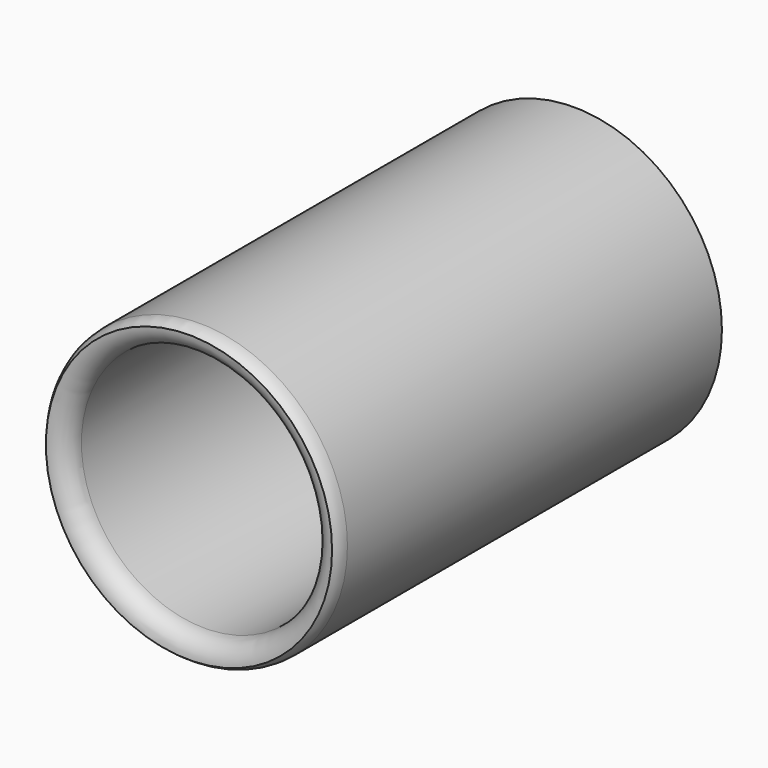
from build123d import *

# Parameters (mm, degrees)
F0_R     = 38.1
F0_R_2   = 31.75
F1_DEPTH = 123.825
F2_R     = 38.1
F3_DEPTH = 6.35
F4_R     = 5.08


# Not quite as in the source:
# - a fillet or chamfer that OpenCascade refuses, or shapes differently, is made with other operations: its cross-section is extruded or revolved along the edge and cut away or added


with BuildPart() as f1:
    # F0 (on Front) → F1 (new body)
    with BuildSketch(Plane.XZ):
        Circle(F0_R)
        Circle(F0_R_2, mode=Mode.SUBTRACT)
    extrude(amount=F1_DEPTH)

    # F2 (on Front) → F3 (join)
    with BuildSketch(Plane.XZ):
        Circle(F2_R)
    extrude(amount=F3_DEPTH)

    # F4
    f4_edges = [f1.edges().sort_by_distance(p)[0] for p in [
        (-31.75, -123.825, 0),
    ]]
    fillet(f4_edges, radius=F4_R)

    # F5: fillet of radius 5.08 on 1 edges, made by hand

    # F5_s1 → F5_t2 (revolve, cut)
    with BuildSketch(Plane.XY):
        with BuildLine():
            ThreePointArc((36.83, -123.825), (37.7719048812, -122.2609470592), (38.1, -120.4648958349))
            Line((38.1, -120.4648958349), (38.1, -123.825))
            Line((38.1, -123.825), (36.83, -123.825))
        make_face()
    revolve(axis=Axis((0, -123.825, 0), (0, -1, 0)), mode=Mode.SUBTRACT)


solid = f1.part
